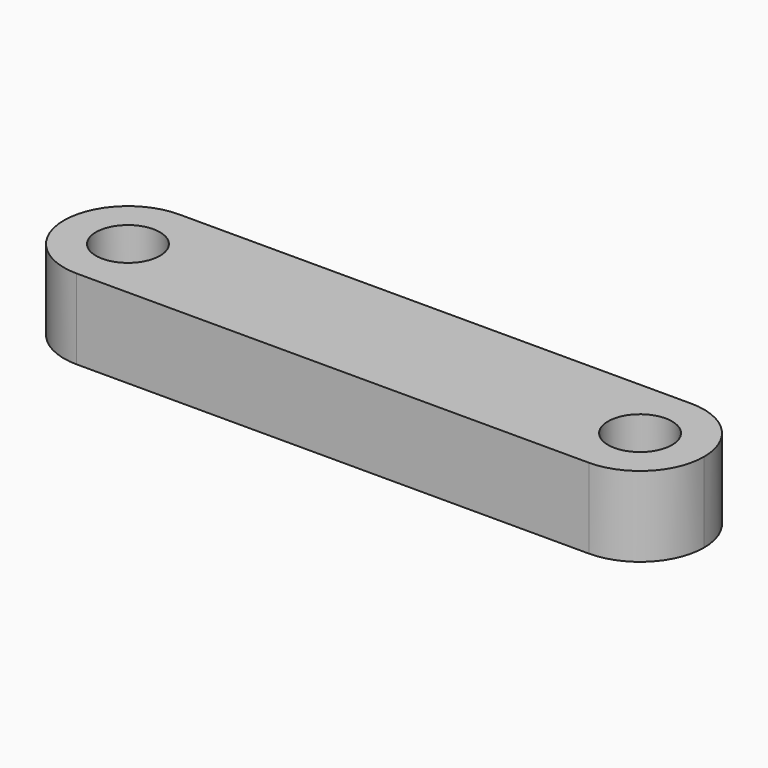
from build123d import *

# Parameters (mm, degrees)
F0_W     = 127
F0_H     = 25.4
F1_DEPTH = 15.875
F2_R     = 6.35
F3_DEPTH = 15.876
F4_R     = 12.69999
F5_R     = 6.35
F6_DEPTH = 15.876
F7_R     = 12.69999


# Not quite as in the source:
# - a fillet or chamfer is up to 0.001 mm smaller than in the source, because OpenCascade refuses the exact size


with BuildPart() as f1:
    # F0 (on Top) → F1 (new body)
    with BuildSketch(Plane.XY):
        with Locations((65.2798527717, 12.1217946971)):
            Rectangle(F0_W, F0_H)
    extrude(amount=F1_DEPTH)

    # F2 (on face) → F3 (cut, through all)
    with BuildSketch(Plane(origin=(0, 0, 0), x_dir=(1, 0, 0), z_dir=(0, 0, -1))):
        with Locations((116.0798527717, -12.1217946971)):
            Circle(F2_R)
    extrude(amount=-F3_DEPTH, mode=Mode.SUBTRACT)

    # F4 (radius 12.7 in the source; OpenCascade refuses exactly that, so slightly less here)
    f4_edges = [f1.edges().sort_by_distance(p)[0] for p in [
        (128.779853, 24.821795, 7.9375),
        (128.779853, -0.578205, 7.9375),
    ]]
    fillet(f4_edges, radius=F4_R)

    # F5 (on face) → F6 (cut, through all)
    with BuildSketch(Plane.XY.offset(15.875)):
        with Locations((14.4798527717, 12.1217946971)):
            Circle(F5_R)
    extrude(amount=-F6_DEPTH, mode=Mode.SUBTRACT)

    # F7 (radius 12.7 in the source; OpenCascade refuses exactly that, so slightly less here)
    f7_edges = [f1.edges().sort_by_distance(p)[0] for p in [
        (1.779853, 24.821795, 7.9375),
        (1.779853, -0.578205, 7.9375),
    ]]
    fillet(f7_edges, radius=F7_R)


solid = f1.part
